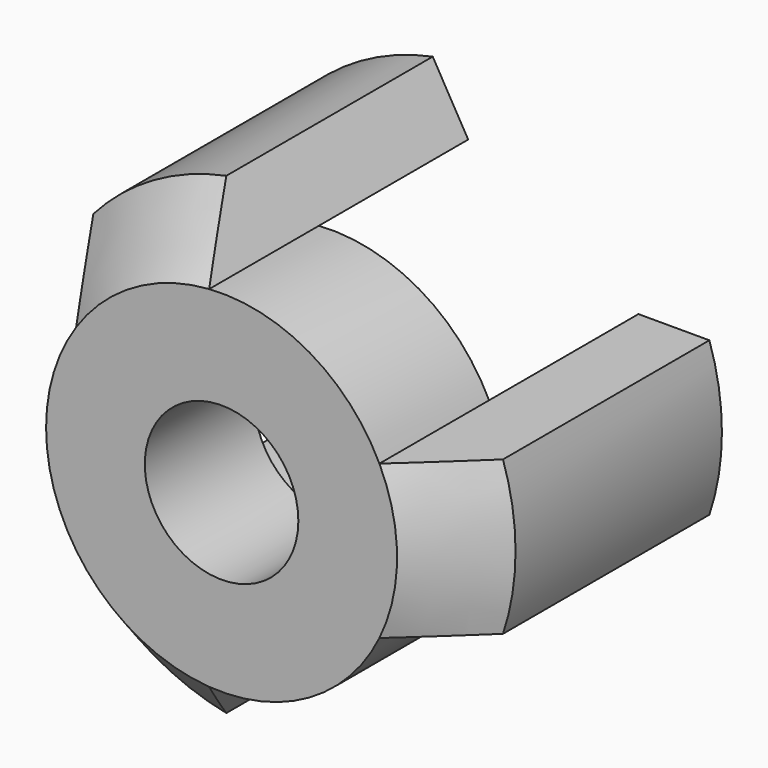
from build123d import *

# Parameters (mm, degrees)
F0_R        = 101.6
F0_R_2      = 44.45
F1_DEPTH    = 79.375
F3_DEPTH    = 187.452
F4_SIZE     = 38.1
F5_T2_ANGLE = 117.4823583848
F6_T2_ANGLE = 117.4823583848


# Not quite as in the source:
# - a fillet or chamfer that OpenCascade refuses, or shapes differently, is made with other operations: its cross-section is extruded or revolved along the edge and cut away or added


with BuildPart() as f1:
    # F0 (on Front) → F1 (new body)
    with BuildSketch(Plane.XZ):
        Circle(F0_R)
        Circle(F0_R_2, mode=Mode.SUBTRACT)
    extrude(amount=F1_DEPTH)

    # F2 (on face) → F3 (join)
    with BuildSketch(Plane.XZ.offset(79.375)):
        with BuildLine():
            Line((132.4397504528, 44.45), (91.3605905191, 44.45))
            ThreePointArc((91.3605905191, 44.45), (101.6, 0), (91.3605905191, -44.45))
            Line((91.3605905191, -44.45), (132.4397504528, -44.45))
            ThreePointArc((132.4397504528, -44.45), (139.7, 0), (132.4397504528, 44.45))
        make_face()
        with BuildLine():
            Line((-104.7147044246, 92.471188363), (-84.1751244578, 56.8955922943))
            ThreePointArc((-84.1751244578, 56.8955922943), (-50.8, 87.9881810245), (-7.1854660613, 101.3455922943))
            Line((-7.1854660613, 101.3455922943), (-27.7250460282, 136.921188363))
            ThreePointArc((-27.7250460282, 136.921188363), (-69.85, 120.9837489087), (-104.7147044246, 92.471188363))
        make_face()
        with BuildLine():
            Line((-27.7250460282, -136.921188363), (-7.1854660613, -101.3455922943))
            ThreePointArc((-7.1854660613, -101.3455922943), (-50.8, -87.9881810245), (-84.1751244578, -56.8955922943))
            Line((-84.1751244578, -56.8955922943), (-104.7147044246, -92.471188363))
            ThreePointArc((-104.7147044246, -92.471188363), (-69.85, -120.9837489087), (-27.7250460282, -136.921188363))
        make_face()
    extrude(amount=-F3_DEPTH)

    # F4
    f4_edges = [f1.edges().sort_by_distance(p)[0] for p in [
        (139.7, -79.375, 0),
    ]]
    chamfer(f4_edges, length=F4_SIZE)

    # F5: chamfer of 38.1 on 1 edges, made by hand

    # F5_s1 → F5_t2 (revolve, cut)
    with BuildSketch(Plane(origin=(0, 0, 0), x_dir=(0, 1, 0), z_dir=(-0.0219688003, 0, 0.9997586568))):
        Polygon((-79.375, 101.6), (-41.275, 139.7), (-79.375, 139.7), align=None)
    revolve(axis=Axis((0, -79.375, 0), (0, -1, 0)), revolution_arc=F5_T2_ANGLE, mode=Mode.SUBTRACT)

    # F6: chamfer of 38.1 on 1 edges, made by hand

    # F6_s1 → F6_t2 (revolve, cut)
    with BuildSketch(Plane(origin=(0, 0, 0), x_dir=(0, 1, 0), z_dir=(0.8768007946, 0, -0.4808537893))):
        Polygon((-79.375, 101.6), (-41.275, 139.7), (-79.375, 139.7), align=None)
    revolve(axis=Axis((0, -79.375, 0), (0, -1, 0)), revolution_arc=F6_T2_ANGLE, mode=Mode.SUBTRACT)


solid = f1.part
